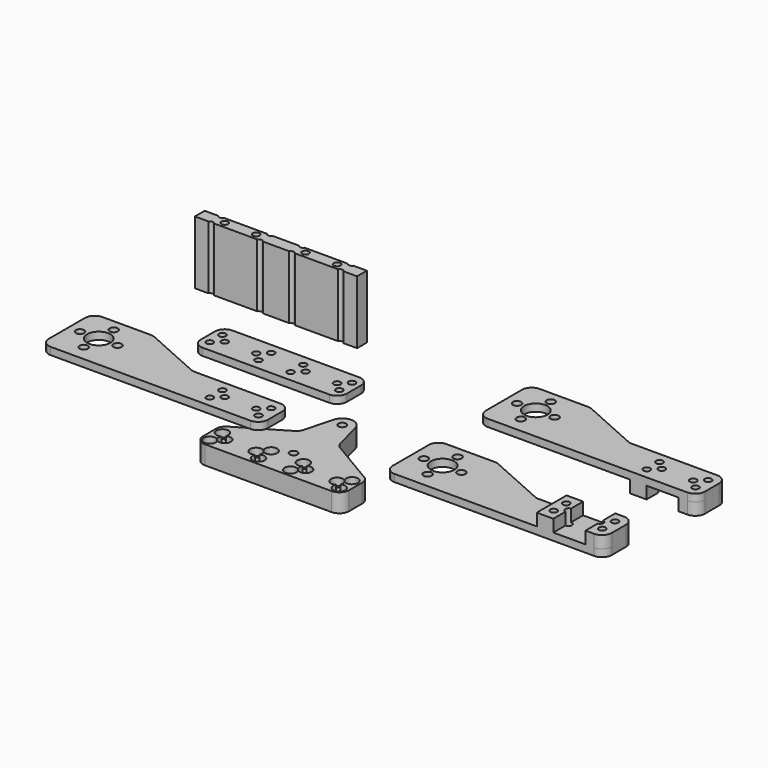
from build123d import *

# Parameters (mm, degrees)
F0_R      = 2.032
F0_R_2    = 1.778
F1_DEPTH  = 9.652
F2_R      = 5.08
F4_R      = 2.159
F4_R_2    = 1.778
F4_R_3    = 6.096
F5_DEPTH  = 3.81
F6_R      = 5.08
F8_R      = 1.778
F9_DEPTH  = 3.81
F10_R     = 5.08
F11_W     = 79.248
F11_H     = 32.512
F12_DEPTH = 6.35
F14_W     = 8.636
F14_H     = 19.431
F14_R     = 1.778
F15_DEPTH = 6.35
F17_R     = 1.778
F17_W     = 8.636
F17_H     = 19.431
F18_DEPTH = 6.35
F19_R     = 1.778
F20_DEPTH = 3.81
F21_R     = 1.778
F22_DEPTH = 140.7849183513
F25_R     = 1.778
F26_DEPTH = 33.02
F27_R     = 1.778
F28_DEPTH = 29.211
F29_R     = 1.778
F30_DEPTH = 83.821


with BuildPart() as f1:
    # F0 (on Top) → F1 (new body)
    with BuildSketch(Plane.XY):
        with BuildLine():
            ThreePointArc((-5.6405441012, 39.0210586621), (-0.7671066942, 31.7087122223), (5.842, 37.5001292613))
            ThreePointArc((5.842, 37.5001292613), (5.791417039, 38.2672359556), (5.6405441012, 39.0210586621))
            ThreePointArc((5.6405441012, 39.0210586621), (0, 43.3421292613), (-5.6405441012, 39.0210586621))
        make_face()
        with Locations((0, 37.5001292613)):
            Circle(F0_R, mode=Mode.SUBTRACT)
        with BuildLine():
            ThreePointArc((5.6405441012, 39.0210586621), (5.791417039, 38.2672359556), (5.842, 37.5001292613))
            ThreePointArc((5.842, 37.5001292613), (-0.7671066942, 31.7087122223), (-5.6405441012, 39.0210586621))
            Line((-5.6405441012, 39.0210586621), (-10.16, 22.2601292613))
            Line((-10.16, 22.2601292613), (10.16, 22.2601292613))
            Line((10.16, 22.2601292613), (5.6405441012, 39.0210586621))
        make_face()
        Polygon((38.1, 5.7501292613), (10.16, 22.2601292613), (-10.16, 22.2601292613), (-38.1, 5.7501292613), (-38.1, -10.7598707387), (38.1, -10.7598707387), align=None)
        with Locations((-33.782, -6.6323707387)):
            Circle(F0_R_2, mode=Mode.SUBTRACT)
        with Locations((-29.2959148749, -2.5048707387)):
            Circle(F0_R_2, mode=Mode.SUBTRACT)
        with Locations((-33.782, 1.6226292613)):
            Circle(F0_R_2, mode=Mode.SUBTRACT)
        with Locations((-8.382, -6.6323707387)):
            Circle(F0_R_2, mode=Mode.SUBTRACT)
        with Locations((-12.8680851251, -2.5048707387)):
            Circle(F0_R_2, mode=Mode.SUBTRACT)
        with Locations((-8.382, 1.6226292613)):
            Circle(F0_R_2, mode=Mode.SUBTRACT)
        with Locations((8.382, -6.6323707387)):
            Circle(F0_R_2, mode=Mode.SUBTRACT)
        with Locations((8.382, 1.6226292613)):
            Circle(F0_R_2, mode=Mode.SUBTRACT)
        with Locations((12.8680851251, -2.5048707387)):
            Circle(F0_R_2, mode=Mode.SUBTRACT)
        with Locations((33.782, -6.6323707387)):
            Circle(F0_R_2, mode=Mode.SUBTRACT)
        with Locations((29.2959148749, -2.5048707387)):
            Circle(F0_R_2, mode=Mode.SUBTRACT)
        with Locations((33.782, 1.6226292613)):
            Circle(F0_R_2, mode=Mode.SUBTRACT)
        with Locations((0, 5.7501292613)):
            Circle(F0_R, mode=Mode.SUBTRACT)
    extrude(amount=F1_DEPTH)

    # F2
    f2_edges = [f1.edges().sort_by_distance(p)[0] for p in [
        (-10.16, 22.260129, 4.826),
        (10.16, 22.260129, 4.826),
        (-38.1, -10.759871, 4.826),
        (38.1, -10.759871, 4.826),
        (38.1, 5.750129, 4.826),
        (-38.1, 5.750129, 4.826),
    ]]
    fillet(f2_edges, radius=F2_R)

    # F19 (on face) → F20 (cut)
    with BuildSketch(Plane.XY.offset(9.652)):
        with BuildLine():
            ThreePointArc((-10.0231154792, -3.9143999913), (-9.6930851251, -2.5048707387), (-10.0231154792, -1.0953414861))
            ThreePointArc((-10.0231154792, -1.0953414861), (-6.0454973307, 3.7723688446), (-11.2269696459, 0.2131000087))
            ThreePointArc((-11.2269696459, 0.2131000087), (-16.0430851251, -2.5048707387), (-11.2269696459, -5.2228414861))
            ThreePointArc((-11.2269696459, -5.2228414861), (-6.0454973307, -8.782110322), (-10.0231154792, -3.9143999913))
        make_face()
        with Locations((-12.8680851251, -2.5048707387)):
            Circle(F19_R, mode=Mode.SUBTRACT)
        with BuildLine():
            ThreePointArc((-30.9370303541, -5.2228414861), (-26.1209148749, -2.5048707387), (-30.9370303541, 0.2131000087))
            ThreePointArc((-30.9370303541, 0.2131000087), (-36.1185026693, 3.7723688446), (-32.1408845208, -1.0953414861))
            ThreePointArc((-32.1408845208, -1.0953414861), (-32.4709148749, -2.5048707387), (-32.1408845208, -3.9143999913))
            ThreePointArc((-32.1408845208, -3.9143999913), (-36.1185026693, -8.782110322), (-30.9370303541, -5.2228414861))
        make_face()
        with Locations((-29.2959148749, -2.5048707387)):
            Circle(F19_R, mode=Mode.SUBTRACT)
        with BuildLine():
            ThreePointArc((32.1408845208, -1.0953414861), (36.1185026693, 3.7723688446), (30.9370303541, 0.2131000087))
            ThreePointArc((30.9370303541, 0.2131000087), (26.1209148749, -2.5048707387), (30.9370303541, -5.2228414861))
            ThreePointArc((30.9370303541, -5.2228414861), (36.1185026693, -8.782110322), (32.1408845208, -3.9143999913))
            ThreePointArc((32.1408845208, -3.9143999913), (32.4709148749, -2.5048707387), (32.1408845208, -1.0953414861))
        make_face()
        with Locations((29.2959148749, -2.5048707387)):
            Circle(F19_R, mode=Mode.SUBTRACT)
        with BuildLine():
            ThreePointArc((11.2269696459, 0.2131000087), (6.0454973307, 3.7723688446), (10.0231154792, -1.0953414861))
            ThreePointArc((10.0231154792, -1.0953414861), (9.6930851251, -2.5048707387), (10.0231154792, -3.9143999913))
            ThreePointArc((10.0231154792, -3.9143999913), (6.0454973307, -8.782110322), (11.2269696459, -5.2228414861))
            ThreePointArc((11.2269696459, -5.2228414861), (16.0430851251, -2.5048707387), (11.2269696459, 0.2131000087))
        make_face()
        with Locations((12.8680851251, -2.5048707387)):
            Circle(F19_R, mode=Mode.SUBTRACT)
    extrude(amount=-F20_DEPTH, mode=Mode.SUBTRACT)


with BuildPart() as f5:
    # F4 (on offset) → F5 (new body)
    with BuildSketch(Plane.XY.offset(25.4)):
        Polygon((-117.348, -12.2203707387), (-3.048, -12.2203707387), (-3.048, 7.2106292613), (-53.848, 7.2106292613), (-85.852, 21.4981292613), (-117.348, 21.4981292613), align=None)
        with Locations((-101.6, -4.0288707387)):
            Circle(F4_R, mode=Mode.SUBTRACT)
        with Locations((-33.782, -6.6323707387)):
            Circle(F4_R_2, mode=Mode.SUBTRACT)
        with Locations((-8.382, -6.6323707387)):
            Circle(F4_R_2, mode=Mode.SUBTRACT)
        with Locations((-33.782, 1.6226292613)):
            Circle(F4_R_2, mode=Mode.SUBTRACT)
        with Locations((-29.2959148749, -2.5048707387)):
            Circle(F4_R_2, mode=Mode.SUBTRACT)
        with Locations((-12.8680851251, -2.5048707387)):
            Circle(F4_R_2, mode=Mode.SUBTRACT)
        with Locations((-8.382, 1.6226292613)):
            Circle(F4_R_2, mode=Mode.SUBTRACT)
        with Locations((-111.379, 5.7501292613)):
            Circle(F4_R, mode=Mode.SUBTRACT)
        with Locations((-101.6, 5.7501292613)):
            Circle(F4_R_3, mode=Mode.SUBTRACT)
        with Locations((-91.821, 5.7501292613)):
            Circle(F4_R, mode=Mode.SUBTRACT)
        with Locations((-101.6, 15.5291292613)):
            Circle(F4_R, mode=Mode.SUBTRACT)
    extrude(amount=F5_DEPTH)

    # F6
    f6_edges = [f5.edges().sort_by_distance(p)[0] for p in [
        (-117.348, 21.498129, 27.305),
        (-117.348, -12.220371, 27.305),
        (-85.852, 21.498129, 27.305),
        (-53.848, 7.210629, 27.305),
        (-3.048, 7.210629, 27.305),
        (-3.048, -12.220371, 27.305),
    ]]
    fillet(f6_edges, radius=F6_R)


with BuildPart() as f9:
    # F8 (on offset) → F9 (new body)
    with BuildSketch(Plane.XY.offset(50.8)):
        Polygon((-38.1, 7.2106292613), (-38.1, 2.851327781), (-38.1, -5.6798707387), (-38.1, -12.2203707387), (38.1, -12.2203707387), (38.1, -5.6798707387), (38.1, 2.851327781), (38.1, 7.2106292613), align=None)
        with Locations((-33.782, -6.6323707387)):
            Circle(F8_R, mode=Mode.SUBTRACT)
        with Locations((-8.382, -6.6323707387)):
            Circle(F8_R, mode=Mode.SUBTRACT)
        with Locations((8.382, -6.6323707387)):
            Circle(F8_R, mode=Mode.SUBTRACT)
        with Locations((33.782, -6.6323707387)):
            Circle(F8_R, mode=Mode.SUBTRACT)
        with Locations((-29.2959148749, -2.5048707387)):
            Circle(F8_R, mode=Mode.SUBTRACT)
        with Locations((-33.782, 1.6226292613)):
            Circle(F8_R, mode=Mode.SUBTRACT)
        with Locations((-12.8680851251, -2.5048707387)):
            Circle(F8_R, mode=Mode.SUBTRACT)
        with Locations((-8.382, 1.6226292613)):
            Circle(F8_R, mode=Mode.SUBTRACT)
        with Locations((12.8680851251, -2.5048707387)):
            Circle(F8_R, mode=Mode.SUBTRACT)
        with Locations((8.382, 1.6226292613)):
            Circle(F8_R, mode=Mode.SUBTRACT)
        with Locations((29.2959148749, -2.5048707387)):
            Circle(F8_R, mode=Mode.SUBTRACT)
        with Locations((33.782, 1.6226292613)):
            Circle(F8_R, mode=Mode.SUBTRACT)
    extrude(amount=F9_DEPTH)

    # F10
    f10_edges = [f9.edges().sort_by_distance(p)[0] for p in [
        (38.1, 7.210629, 52.705),
        (38.1, -12.220371, 52.705),
        (-38.1, 7.210629, 52.705),
        (-38.1, -12.220371, 52.705),
    ]]
    fillet(f10_edges, radius=F10_R)


with BuildPart() as f12:
    # F11 (on Top) → F12 (new body)
    with BuildSketch(Plane.XY):
        with Locations((-39.624, -41.30778909)):
            Rectangle(F11_W, F11_H)
    extrude(amount=F12_DEPTH)

    # F21 (on face) → F22 (cut, through all)
    with BuildSketch(Plane.XZ.offset(57.56378909)):
        with Locations((-68.326, 3.175)):
            Circle(F21_R)
        with Locations((-53.086, 3.175)):
            Circle(F21_R)
        with Locations((-10.922, 3.175)):
            Circle(F21_R)
        with Locations((-26.162, 3.175)):
            Circle(F21_R)
    extrude(amount=-F22_DEPTH, mode=Mode.SUBTRACT)


with BuildPart() as f13_1:
    # F13: copy of F5
    add(f5.part.moved(Location((179.324, 0, 0))))

    # F14 (on face) → F15 (join)
    with BuildSketch(Plane.XY.offset(29.21)):
        with Locations((145.542, -2.5048707387)):
            Rectangle(F14_W, F14_H)
        with Locations((145.542, -6.6323707387)):
            Circle(F14_R, mode=Mode.SUBTRACT)
        with Locations((145.542, 1.6226292613)):
            Circle(F14_R, mode=Mode.SUBTRACT)
        with BuildLine():
            Line((171.196, 7.2106292613), (166.624, 7.2106292613))
            Line((166.624, 7.2106292613), (166.624, -12.2203707387))
            Line((166.624, -12.2203707387), (171.196, -12.2203707387))
            ThreePointArc((171.196, -12.2203707387), (174.7881024484, -10.7324731871), (176.276, -7.1403707387))
            Line((176.276, -7.1403707387), (176.276, 2.1306292613))
            ThreePointArc((176.276, 2.1306292613), (174.7881024484, 5.7227317097), (171.196, 7.2106292613))
        make_face()
        with Locations((170.942, -6.6323707387)):
            Circle(F14_R, mode=Mode.SUBTRACT)
        with Locations((170.942, 1.6226292613)):
            Circle(F14_R, mode=Mode.SUBTRACT)
    extrude(amount=F15_DEPTH)

    # F29 (on face) → F30 (cut, through all)
    with BuildSketch(Plane(origin=(0, 0, 25.4), x_dir=(1, 0, 0), z_dir=(0, 0, -1))):
        with Locations((166.4559148749, 2.5048707387)):
            Circle(F29_R)
        with Locations((150.0280851251, 2.5048707387)):
            Circle(F29_R)
    extrude(amount=-F30_DEPTH, mode=Mode.SUBTRACT)


with BuildPart() as f16_1:
    # F16: copy of F5
    add(f5.part.moved(Location((178.562, 61.722, 0))))

    # F17 (on face) → F18 (join)
    with BuildSketch(Plane(origin=(0, 0, 25.4), x_dir=(1, 0, 0), z_dir=(0, 0, -1))):
        with BuildLine():
            Line((165.862, -68.9326292613), (170.434, -68.9326292613))
            ThreePointArc((170.434, -68.9326292613), (174.0261024484, -67.4447317097), (175.514, -63.8526292613))
            Line((175.514, -63.8526292613), (175.514, -54.5816292613))
            ThreePointArc((175.514, -54.5816292613), (174.0261024484, -50.9895268129), (170.434, -49.5016292613))
            Line((170.434, -49.5016292613), (165.862, -49.5016292613))
            Line((165.862, -49.5016292613), (165.862, -68.9326292613))
        make_face()
        with Locations((170.18, -63.3446292613)):
            Circle(F17_R, mode=Mode.SUBTRACT)
        with Locations((170.18, -55.0896292613)):
            Circle(F17_R, mode=Mode.SUBTRACT)
        with Locations((144.78, -59.2171292613)):
            Rectangle(F17_W, F17_H)
        with Locations((144.78, -63.3446292613)):
            Circle(F17_R, mode=Mode.SUBTRACT)
        with Locations((144.78, -55.0896292613)):
            Circle(F17_R, mode=Mode.SUBTRACT)
    extrude(amount=F18_DEPTH)

    # F27 (on face) → F28 (cut, through all)
    with BuildSketch(Plane.XY.offset(29.21)):
        with Locations((149.2660851251, 59.2171292613)):
            Circle(F27_R)
        with Locations((165.6939148749, 59.2171292613)):
            Circle(F27_R)
    extrude(amount=-F28_DEPTH, mode=Mode.SUBTRACT)


with BuildPart() as f26:
    # F25 (on offset) → F26 (new body)
    with BuildSketch(Plane.XY.offset(76.2)):
        with BuildLine():
            Line((35.283341983, -5.6798707387), (42.2842092812, -5.6798707387))
            Line((42.2842092812, -5.6798707387), (42.2842092812, 0.6701292613))
            Line((42.2842092812, 0.6701292613), (35.283341983, 0.6701292613))
            ThreePointArc((35.283341983, 0.6701292613), (33.782, -0.1553707387), (32.280658017, 0.6701292613))
            Line((32.280658017, 0.6701292613), (9.883341983, 0.6701292613))
            ThreePointArc((9.883341983, 0.6701292613), (8.382, -0.1553707387), (6.880658017, 0.6701292613))
            Line((6.880658017, 0.6701292613), (-6.880658017, 0.6701292613))
            ThreePointArc((-6.880658017, 0.6701292613), (-8.382, -0.1553707387), (-9.883341983, 0.6701292613))
            Line((-9.883341983, 0.6701292613), (-32.280658017, 0.6701292613))
            ThreePointArc((-32.280658017, 0.6701292613), (-33.782, -0.1553707387), (-35.283341983, 0.6701292613))
            Line((-35.283341983, 0.6701292613), (-42.2842092812, 0.6701292613))
            Line((-42.2842092812, 0.6701292613), (-42.2842092812, -5.6798707387))
            Line((-42.2842092812, -5.6798707387), (-35.283341983, -5.6798707387))
            ThreePointArc((-35.283341983, -5.6798707387), (-33.782, -4.8543707387), (-32.280658017, -5.6798707387))
            Line((-32.280658017, -5.6798707387), (-9.883341983, -5.6798707387))
            ThreePointArc((-9.883341983, -5.6798707387), (-8.382, -4.8543707387), (-6.880658017, -5.6798707387))
            Line((-6.880658017, -5.6798707387), (6.880658017, -5.6798707387))
            ThreePointArc((6.880658017, -5.6798707387), (8.382, -4.8543707387), (9.883341983, -5.6798707387))
            Line((9.883341983, -5.6798707387), (32.280658017, -5.6798707387))
            ThreePointArc((32.280658017, -5.6798707387), (33.782, -4.8543707387), (35.283341983, -5.6798707387))
        make_face()
        with Locations((-29.2959148749, -2.5048707387)):
            Circle(F25_R, mode=Mode.SUBTRACT)
        with Locations((-12.8680851251, -2.5048707387)):
            Circle(F25_R, mode=Mode.SUBTRACT)
        with Locations((12.8680851251, -2.5048707387)):
            Circle(F25_R, mode=Mode.SUBTRACT)
        with Locations((29.2959148749, -2.5048707387)):
            Circle(F25_R, mode=Mode.SUBTRACT)
    extrude(amount=F26_DEPTH)


solid = Compound([f1.part, f5.part, f9.part, f13_1.part, f16_1.part, f26.part])
